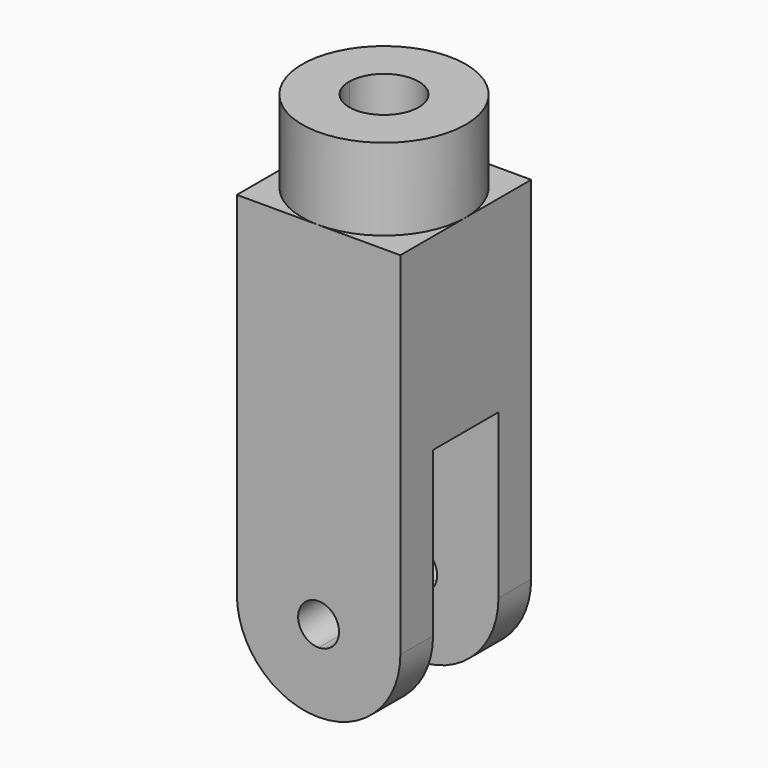
from build123d import *

# Parameters (mm, degrees)
F0_R     = 10
F0_R_2   = 4.25
F1_DEPTH = 10
F3_DEPTH = 53
F5_DEPTH = 25
F6_DEPTH = 23
F7_R     = 9.99999
F8_D     = 8.5


# Not quite as in the source:
# - a fillet or chamfer is up to 0.001 mm smaller than in the source, because OpenCascade refuses the exact size
# - a feature names something its author has since deleted; it is built from what else it names


with BuildPart() as f1:
    # F0 (on Top) → F1 (new body)
    with BuildSketch(Plane.XY):
        Circle(F0_R)
        Circle(F0_R_2, mode=Mode.SUBTRACT)
    extrude(amount=F1_DEPTH)

    # F2 (on face) → F3 (join)
    with BuildSketch(Plane.XY):
        with BuildLine():
            ThreePointArc((8.6602540378, -5), (5, -8.6602540378), (0, -10))
            Line((0, -10), (10, -10))
            Line((10, -10), (10, -5))
            Line((10, -5), (8.6602540378, -5))
        make_face()
        with BuildLine():
            ThreePointArc((-8.6602540378, -5), (-5, -8.6602540378), (0, -10))
            ThreePointArc((0, -10), (5, -8.6602540378), (8.6602540378, -5))
            Line((8.6602540378, -5), (-8.6602540378, -5))
        make_face()
        with BuildLine():
            Line((-10, -10), (0, -10))
            ThreePointArc((0, -10), (-5, -8.6602540378), (-8.6602540378, -5))
            Line((-8.6602540378, -5), (-10, -5))
            Line((-10, -5), (-10, -10))
        make_face()
        with BuildLine():
            Line((8.6602540378, 5), (10, 5))
            Line((10, 5), (10, 10))
            Line((10, 10), (-2.67e-08, 10))
            ThreePointArc((-2.67e-08, 10), (4.9999999884, 8.6602540445), (8.6602540378, 5))
        make_face()
        with BuildLine():
            Line((-10, 10), (-10, 5))
            Line((-10, 5), (-8.6602540378, 5))
            ThreePointArc((-8.6602540378, 5), (-5.0000000116, 8.6602540312), (-2.67e-08, 10))
            Line((-2.67e-08, 10), (-10, 10))
        make_face()
        with BuildLine():
            ThreePointArc((-2.67e-08, 10), (-5.0000000116, 8.6602540312), (-8.6602540378, 5))
            Line((-8.6602540378, 5), (8.6602540378, 5))
            ThreePointArc((8.6602540378, 5), (4.9999999884, 8.6602540445), (-2.67e-08, 10))
        make_face()
    extrude(amount=-F3_DEPTH)

    # F4 (on face) → F5 (cut)
    with BuildSketch(Plane.XZ.offset(10)):
        with BuildLine():
            ThreePointArc((2.5, -43), (-1.767766953, -41.232233047), (0, -45.5))
            ThreePointArc((0, -45.5), (1.767766953, -44.767766953), (2.5, -43))
        make_face()
    extrude(amount=-F5_DEPTH, mode=Mode.SUBTRACT)

    # F2 (on face) → F6 (join)
    with BuildSketch(Plane.XY):
        with BuildLine():
            ThreePointArc((4.25, 0), (0, 4.25), (-4.25, 0))
            Line((-4.25, 0), (4.25, 0))
        make_face()
        with BuildLine():
            ThreePointArc((-10, 0), (-9.6592582629, -2.588190451), (-8.6602540378, -5))
            Line((-8.6602540378, -5), (8.6602540378, -5))
            ThreePointArc((8.6602540378, -5), (9.6592582629, -2.588190451), (10, 0))
            Line((10, 0), (4.25, 0))
            ThreePointArc((4.25, 0), (0, -4.25), (-4.25, 0))
            Line((-4.25, 0), (-10, 0))
        make_face()
        with BuildLine():
            ThreePointArc((-8.6602540378, 5), (-9.6592582629, 2.588190451), (-10, 0))
            Line((-10, 0), (-4.25, 0))
            ThreePointArc((-4.25, 0), (0, 4.25), (4.25, 0))
            Line((4.25, 0), (10, 0))
            ThreePointArc((10, 0), (9.6592582629, 2.588190451), (8.6602540378, 5))
            Line((8.6602540378, 5), (-8.6602540378, 5))
        make_face()
        with BuildLine():
            Line((-10, 5), (-10, 0))
            ThreePointArc((-10, 0), (-9.6592582629, 2.588190451), (-8.6602540378, 5))
            Line((-8.6602540378, 5), (-10, 5))
        make_face()
        with BuildLine():
            Line((-10, -5), (-8.6602540378, -5))
            ThreePointArc((-8.6602540378, -5), (-9.6592582629, -2.588190451), (-10, 0))
            Line((-10, 0), (-10, -5))
        make_face()
        with BuildLine():
            ThreePointArc((8.6602540378, 5), (9.6592582629, 2.588190451), (10, 0))
            Line((10, 0), (10, 5))
            Line((10, 5), (8.6602540378, 5))
        make_face()
        with BuildLine():
            ThreePointArc((10, 0), (9.6592582629, -2.588190451), (8.6602540378, -5))
            Line((8.6602540378, -5), (10, -5))
            Line((10, -5), (10, 0))
        make_face()
        with BuildLine():
            Line((4.25, 0), (-4.25, 0))
            ThreePointArc((-4.25, 0), (0, -4.25), (4.25, 0))
        make_face()
    extrude(amount=-F6_DEPTH)

    # F7 (radius 10 in the source; OpenCascade refuses exactly that, so slightly less here)
    f7_edges = [f1.edges().sort_by_distance(p)[0] for p in [
        (-10, -7.5, -53),
        (-10, 7.5, -53),
        (10, 7.5, -53),
        (10, -7.5, -53),
    ]]
    fillet(f7_edges, radius=F7_R)

    # F8 (through all)
    with Locations(Plane.XY):
        with Locations((0, 0)):
            Hole(F8_D / 2)


solid = f1.part
